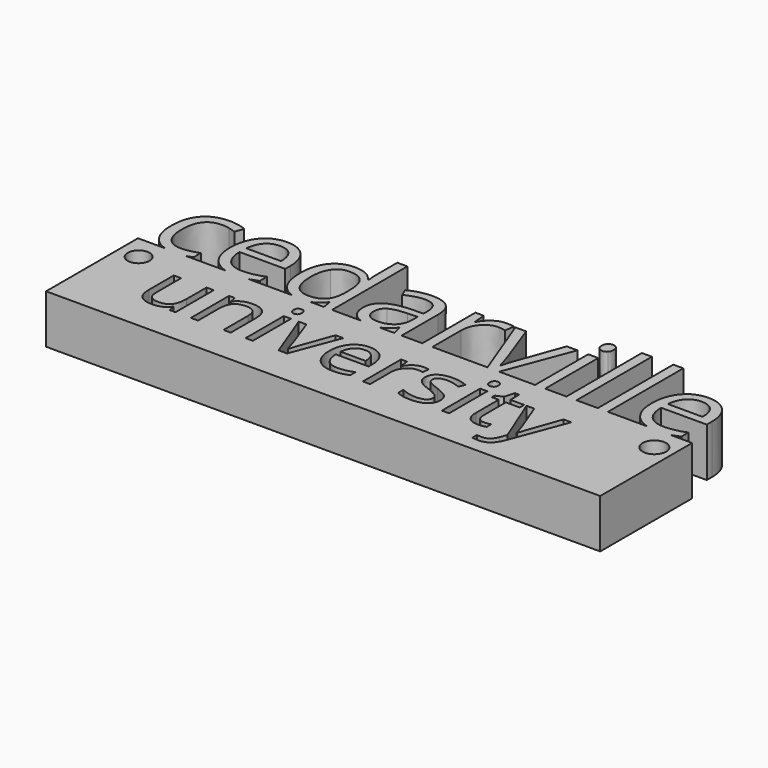
from build123d import *

# Parameters (mm, degrees)
F0_W         = 2.6162547147
F0_H         = 17.2652647355
F0_H_2       = 24.5141554478
F1_DEPTH     = 12.7
F2_R         = 2.841361974
F2_R_2       = 3.060651004
F3_DEPTH     = 25.4
F4_TEXT_SIZE = 23.2007315386
F5_DEPTH     = 72.644


# Not quite as in the source:
# - Text() gives the source's letters only with a copy of the font that has no kerning and outlines rounded to 1/6400 em; it was checked with that copy


with BuildPart() as f1:
    # F0 (on Top) → F1 (new body)
    with BuildSketch(Plane.XY):
        with BuildLine():
            Line((-23.2760247454, 28.446094293), (-22.9281989741, 26.1322967708))
            Line((-22.9281989741, 26.1322967708), (-20.8009167206, 26.1322967708))
            Line((-20.8009167206, 26.1322967708), (-20.8009167206, 50.6464522186))
            Line((-20.8009167206, 50.6464522186), (-23.4171714352, 50.6464522186))
            Line((-23.4171714352, 50.6464522186), (-23.4171714352, 43.6193634475))
            Line((-23.4171714352, 43.6193634475), (-23.3516390435, 42.4044937245))
            Line((-23.3516390435, 42.4044937245), (-23.240738073, 41.1593782822))
            Line((-23.240738073, 41.1593782822), (-23.4474171545, 41.1593782822))
            add(Edge.make_bspline(
                [(-28.8361961332, 43.7151415584), (-25.3226517477, 43.7151415584), (-23.4474171545, 41.1593782822)],
                knots=[0, 0, 0, 1, 1, 1], degree=2))
            add(Edge.make_bspline(
                [(-34.0989512818, 41.3509345041), (-32.208593829, 43.7151415584), (-28.8361961332, 43.7151415584)],
                knots=[0, 0, 0, 1, 1, 1], degree=2))
            add(Edge.make_bspline(
                [(-35.9893087346, 34.7170400831), (-35.9893087346, 38.9867274498), (-34.0989512818, 41.3509345041)],
                knots=[0, 0, 0, 1, 1, 1], degree=2))
            add(Edge.make_bspline(
                [(-34.1065127116, 28.1310347176), (-35.9893087346, 30.4473527164), (-35.9893087346, 34.7170400831)],
                knots=[0, 0, 0, 1, 1, 1], degree=2))
            add(Edge.make_bspline(
                [(-31.138536455, 26.1322967708), (-32.9208740045, 26.6723975397), (-34.1065127116, 28.1310347176)],
                knots=[0.3702776654, 0.3702776654, 0.3702776654, 1, 1, 1], degree=2))
            Line((-31.138536455, 26.1322967708), (-26.5456043362, 26.1322967708))
            add(Edge.make_bspline(
                [(-23.4171714352, 28.446094293), (-24.5981755511, 26.7288682527), (-26.5456043362, 26.1322967708)],
                knots=[0, 0, 0, 0.6525958331, 0.6525958331, 0.6525958331], degree=2))
            Line((-23.4171714352, 28.446094293), (-23.2760247454, 28.446094293))
        make_face()
        with BuildLine():
            add(Edge.make_bspline(
                [(-28.5034932216, 28.007531364), (-25.8267470684, 28.007531364), (-24.6219592518, 29.4643668409)],
                knots=[0, 0, 0, 1, 1, 1], degree=2))
            add(Edge.make_bspline(
                [(-32.0649266626, 29.6937302119), (-30.8525774162, 28.007531364), (-28.5034932216, 28.007531364)],
                knots=[0, 0, 0, 1, 1, 1], degree=2))
            add(Edge.make_bspline(
                [(-33.277275909, 34.6867943639), (-33.277275909, 31.3799290598), (-32.0649266626, 29.6937302119)],
                knots=[0, 0, 0, 1, 1, 1], degree=2))
            add(Edge.make_bspline(
                [(-32.0573652328, 39.7353090011), (-33.277275909, 37.9482910891), (-33.277275909, 34.6867943639)],
                knots=[0, 0, 0, 1, 1, 1], degree=2))
            add(Edge.make_bspline(
                [(-28.5337389408, 41.5223269132), (-30.8374545566, 41.5223269132), (-32.0573652328, 39.7353090011)],
                knots=[0, 0, 0, 1, 1, 1], degree=2))
            add(Edge.make_bspline(
                [(-24.6370821114, 39.9545904656), (-25.8569927876, 41.5223269132), (-28.5337389408, 41.5223269132)],
                knots=[0, 0, 0, 1, 1, 1], degree=2))
            add(Edge.make_bspline(
                [(-23.4171714352, 34.7170400831), (-23.4171714352, 38.3868540181), (-24.6370821114, 39.9545904656)],
                knots=[0, 0, 0, 1, 1, 1], degree=2))
            Line((-23.4171714352, 34.7170400831), (-23.4171714352, 34.1675761835))
            add(Edge.make_bspline(
                [(-24.6219592518, 29.4643668409), (-23.4171714352, 30.9212023179), (-23.4171714352, 34.1675761835)],
                knots=[0, 0, 0, 1, 1, 1], degree=2))
        make_face(mode=Mode.SUBTRACT)
        with BuildLine():
            Line((-20.8009167206, 26.1322967708), (-22.9281989741, 26.1322967708))
            Line((-22.9281989741, 26.1322967708), (-26.5456043362, 26.1322967708))
            add(Edge.make_bspline(
                [(-26.5456043362, 26.1322967708), (-27.5823024583, 25.8147167187), (-28.8361961332, 25.8147167187)],
                knots=[0.6525958331, 0.6525958331, 0.6525958331, 1, 1, 1], degree=2))
            add(Edge.make_bspline(
                [(-28.8361961332, 25.8147167187), (-30.0905193361, 25.8147167187), (-31.138536455, 26.1322967708)],
                knots=[0, 0, 0, 0.3702776654, 0.3702776654, 0.3702776654], degree=2))
            Line((-31.138536455, 26.1322967708), (-42.60280741, 26.1322967708))
            add(Edge.make_bspline(
                [(-42.60280741, 26.1322967708), (-42.7271751485, 26.1029250075), (-42.85004605, 26.0768462855)],
                knots=[0.9005120931, 0.9005120931, 0.9005120931, 1, 1, 1], degree=2))
            add(Edge.make_bspline(
                [(-42.85004605, 26.0768462855), (-44.0850795858, 25.8147167187), (-45.8342903488, 25.8147167187)],
                knots=[0, 0, 0, 1, 1, 1], degree=2))
            add(Edge.make_bspline(
                [(-45.8342903488, 25.8147167187), (-47.2456387033, 25.8147167187), (-48.4378362443, 26.1322967708)],
                knots=[0, 0, 0, 0.3688754729, 0.3688754729, 0.3688754729], degree=2))
            Line((-48.4378362443, 26.1322967708), (-58.7826764594, 26.1322967708))
            add(Edge.make_bspline(
                [(-58.7826764594, 26.1322967708), (-60.0261827647, 25.8147167187), (-61.5872691221, 25.8147167187)],
                knots=[0.406741787, 0.406741787, 0.406741787, 1, 1, 1], degree=2))
            add(Edge.make_bspline(
                [(-61.5872691221, 25.8147167187), (-62.9782563342, 25.8147167187), (-64.1362590541, 26.1322967708)],
                knots=[0, 0, 0, 0.3708835197, 0.3708835197, 0.3708835197], degree=2))
            Line((-64.1362590541, 26.1322967708), (-71.2608583272, 26.1322967708))
            Line((-71.2608583272, 26.1322967708), (-71.2608583272, -3.7426400431))
            Line((-71.2608583272, -3.7426400431), (72.8596820975, -3.7426400431))
            Line((72.8596820975, -3.7426400431), (72.8596820975, 26.1322967708))
            Line((72.8596820975, 26.1322967708), (67.0278429456, 26.1322967708))
            add(Edge.make_bspline(
                [(67.0278429456, 26.1322967708), (66.9034752071, 26.1029250075), (66.7806043057, 26.0768462855)],
                knots=[0.9005120931, 0.9005120931, 0.9005120931, 1, 1, 1], degree=2))
            add(Edge.make_bspline(
                [(66.7806043057, 26.0768462855), (65.5455707699, 25.8147167187), (63.7963600069, 25.8147167187)],
                knots=[0, 0, 0, 1, 1, 1], degree=2))
            add(Edge.make_bspline(
                [(63.7963600069, 25.8147167187), (62.3850116524, 25.8147167187), (61.1928141113, 26.1322967708)],
                knots=[0, 0, 0, 0.3688754729, 0.3688754729, 0.3688754729], degree=2))
            Line((61.1928141113, 26.1322967708), (50.9570521875, 26.1322967708))
            Line((50.9570521875, 26.1322967708), (48.3407974728, 26.1322967708))
            Line((48.3407974728, 26.1322967708), (42.7957489446, 26.1322967708))
            Line((42.7957489446, 26.1322967708), (40.17949423, 26.1322967708))
            Line((40.17949423, 26.1322967708), (34.6344457018, 26.1322967708))
            Line((34.6344457018, 26.1322967708), (32.0181909871, 26.1322967708))
            Line((32.0181909871, 26.1322967708), (22.6924275533, 26.1322967708))
            Line((22.6924275533, 26.1322967708), (19.6376099096, 26.1322967708))
            Line((19.6376099096, 26.1322967708), (5.3011389876, 26.1322967708))
            Line((5.3011389876, 26.1322967708), (2.6848842729, 26.1322967708))
            Line((2.6848842729, 26.1322967708), (-2.6988537526, 26.1322967708))
            Line((-2.6988537526, 26.1322967708), (-4.6396207375, 26.1322967708))
            Line((-4.6396207375, 26.1322967708), (-8.5637145698, 26.1322967708))
            add(Edge.make_bspline(
                [(-8.5637145698, 26.1322967708), (-9.6384567354, 25.8147167187), (-11.066836077, 25.8147167187)],
                knots=[0.2582329607, 0.2582329607, 0.2582329607, 1, 1, 1], degree=2))
            add(Edge.make_bspline(
                [(-11.066836077, 25.8147167187), (-12.3226429307, 25.8147167187), (-13.3127934671, 26.1322967708)],
                knots=[0, 0, 0, 0.4894320446, 0.4894320446, 0.4894320446], degree=2))
            Line((-13.3127934671, 26.1322967708), (-20.8009167206, 26.1322967708))
        make_face()
        with BuildLine():
            add(Edge.make_bspline(
                [(-26.5456043362, 26.1322967708), (-27.5823024583, 25.8147167187), (-28.8361961332, 25.8147167187)],
                knots=[0.6525958331, 0.6525958331, 0.6525958331, 1, 1, 1], degree=2))
            Line((-26.5456043362, 26.1322967708), (-31.138536455, 26.1322967708))
            add(Edge.make_bspline(
                [(-28.8361961332, 25.8147167187), (-30.0905193361, 25.8147167187), (-31.138536455, 26.1322967708)],
                knots=[0, 0, 0, 0.3702776654, 0.3702776654, 0.3702776654], degree=2))
        make_face()
        with BuildLine():
            add(Edge.make_bspline(
                [(-13.3127934671, 26.1322967708), (-14.3457032256, 26.4635913799), (-15.0895167365, 27.1404874123)],
                knots=[0.4894320446, 0.4894320446, 0.4894320446, 1, 1, 1], degree=2))
            Line((-13.3127934671, 26.1322967708), (-8.5637145698, 26.1322967708))
            add(Edge.make_bspline(
                [(-7.8582693604, 26.391905861), (-8.1895622595, 26.2428565999), (-8.5637145698, 26.1322967708)],
                knots=[0, 0, 0, 0.2582329607, 0.2582329607, 0.2582329607], degree=2))
            add(Edge.make_bspline(
                [(-5.284862748, 28.592281936), (-6.5753467691, 26.9690950032), (-7.8582693604, 26.391905861)],
                knots=[0, 0, 0, 1, 1, 1], degree=2))
            Line((-5.284862748, 28.592281936), (-5.1588389179, 28.592281936))
            Line((-5.1588389179, 28.592281936), (-4.6396207375, 26.1322967708))
            Line((-4.6396207375, 26.1322967708), (-2.6988537526, 26.1322967708))
            Line((-2.6988537526, 26.1322967708), (-2.6988537526, 37.9180453698))
            add(Edge.make_bspline(
                [(-4.1884554254, 42.3112360901), (-2.6988537526, 40.9426172943), (-2.6988537526, 37.9180453698)],
                knots=[0, 0, 0, 1, 1, 1], degree=2))
            add(Edge.make_bspline(
                [(-8.7631204612, 43.6798548859), (-5.6780570982, 43.6798548859), (-4.1884554254, 42.3112360901)],
                knots=[0, 0, 0, 1, 1, 1], degree=2))
            add(Edge.make_bspline(
                [(-11.8154176283, 43.2866605358), (-10.2955702362, 43.6798548859), (-8.7631204612, 43.6798548859)],
                knots=[0, 0, 0, 1, 1, 1], degree=2))
            add(Edge.make_bspline(
                [(-14.6106261818, 42.2028555962), (-13.3352650203, 42.8934661856), (-11.8154176283, 43.2866605358)],
                knots=[0, 0, 0, 1, 1, 1], degree=2))
            Line((-14.6106261818, 42.2028555962), (-13.8040736686, 40.2015971728))
            add(Edge.make_bspline(
                [(-8.9244309638, 41.5223269132), (-11.0819589366, 41.5223269132), (-13.8040736686, 40.2015971728)],
                knots=[0, 0, 0, 1, 1, 1], degree=2))
            add(Edge.make_bspline(
                [(-6.1267019337, 40.5544638973), (-6.9987868386, 41.5223269132), (-8.9244309638, 41.5223269132)],
                knots=[0, 0, 0, 1, 1, 1], degree=2))
            add(Edge.make_bspline(
                [(-5.2546170288, 37.5550967389), (-5.2546170288, 39.5866008815), (-6.1267019337, 40.5544638973)],
                knots=[0, 0, 0, 1, 1, 1], degree=2))
            Line((-5.2546170288, 37.5550967389), (-5.2546170288, 36.4813737057))
            Line((-5.2546170288, 36.4813737057), (-8.1834108423, 36.3855955948))
            add(Edge.make_bspline(
                [(-16.5463522135, 30.9060794583), (-16.5463522135, 36.1335479344), (-8.1834108423, 36.3855955948)],
                knots=[0, 0, 0, 1, 1, 1], degree=2))
            add(Edge.make_bspline(
                [(-15.0895167365, 27.1404874123), (-16.5463522135, 28.4662581059), (-16.5463522135, 30.9060794583)],
                knots=[0, 0, 0, 1, 1, 1], degree=2))
        make_face()
        with BuildLine():
            add(Edge.make_bspline(
                [(-10.5476178966, 27.9772856447), (-8.102755591, 27.9772856447), (-6.7089320291, 29.3156587213)],
                knots=[0, 0, 0, 1, 1, 1], degree=2))
            add(Edge.make_bspline(
                [(-12.9471116234, 28.7157852896), (-12.0901495781, 27.9772856447), (-10.5476178966, 27.9772856447)],
                knots=[0, 0, 0, 1, 1, 1], degree=2))
            add(Edge.make_bspline(
                [(-13.8040736686, 30.875833739), (-13.8040736686, 29.4542849345), (-12.9471116234, 28.7157852896)],
                knots=[0, 0, 0, 1, 1, 1], degree=2))
            add(Edge.make_bspline(
                [(-12.427893443, 33.5450184624), (-13.8040736686, 32.6855359405), (-13.8040736686, 30.875833739)],
                knots=[0, 0, 0, 1, 1, 1], degree=2))
            add(Edge.make_bspline(
                [(-7.9313631819, 34.5154019548), (-11.0517132174, 34.4045009842), (-12.427893443, 33.5450184624)],
                knots=[0, 0, 0, 1, 1, 1], degree=2))
            Line((-7.9313631819, 34.5154019548), (-5.3151084673, 34.6212619722))
            Line((-5.3151084673, 34.6212619722), (-5.3151084673, 33.0636074311))
            add(Edge.make_bspline(
                [(-6.7089320291, 29.3156587213), (-5.3151084673, 30.6540317979), (-5.3151084673, 33.0636074311)],
                knots=[0, 0, 0, 1, 1, 1], degree=2))
        make_face(mode=Mode.SUBTRACT)
        with BuildLine():
            Line((-8.5637145698, 26.1322967708), (-13.3127934671, 26.1322967708))
            add(Edge.make_bspline(
                [(-11.066836077, 25.8147167187), (-12.3226429307, 25.8147167187), (-13.3127934671, 26.1322967708)],
                knots=[0, 0, 0, 0.4894320446, 0.4894320446, 0.4894320446], degree=2))
            add(Edge.make_bspline(
                [(-8.5637145698, 26.1322967708), (-9.6384567354, 25.8147167187), (-11.066836077, 25.8147167187)],
                knots=[0.2582329607, 0.2582329607, 0.2582329607, 1, 1, 1], degree=2))
        make_face()
        with BuildLine():
            add(Edge.make_bspline(
                [(-42.60280741, 26.1322967708), (-42.7271751485, 26.1029250075), (-42.85004605, 26.0768462855)],
                knots=[0.9005120931, 0.9005120931, 0.9005120931, 1, 1, 1], degree=2))
            Line((-42.60280741, 26.1322967708), (-48.4378362443, 26.1322967708))
            add(Edge.make_bspline(
                [(-45.8342903488, 25.8147167187), (-47.2456387033, 25.8147167187), (-48.4378362443, 26.1322967708)],
                knots=[0, 0, 0, 0.3688754729, 0.3688754729, 0.3688754729], degree=2))
            add(Edge.make_bspline(
                [(-42.85004605, 26.0768462855), (-44.0850795858, 25.8147167187), (-45.8342903488, 25.8147167187)],
                knots=[0, 0, 0, 1, 1, 1], degree=2))
        make_face()
        with BuildLine():
            Line((-48.4378362443, 26.1322967708), (-42.60280741, 26.1322967708))
            add(Edge.make_bspline(
                [(-40.2287503821, 26.9338083308), (-41.4770961962, 26.3981544906), (-42.60280741, 26.1322967708)],
                knots=[0, 0, 0, 0.9005120931, 0.9005120931, 0.9005120931], degree=2))
            Line((-40.2287503821, 26.9338083308), (-40.2287503821, 29.2677696658))
            add(Edge.make_bspline(
                [(-45.7385122378, 28.1033094749), (-42.9508651141, 28.1033094749), (-40.2287503821, 29.2677696658)],
                knots=[0, 0, 0, 1, 1, 1], degree=2))
            add(Edge.make_bspline(
                [(-49.8418481487, 29.6786073523), (-48.3850126717, 28.1033094749), (-45.7385122378, 28.1033094749)],
                knots=[0, 0, 0, 1, 1, 1], degree=2))
            add(Edge.make_bspline(
                [(-51.379338877, 34.2936000137), (-51.2986836256, 31.2539052296), (-49.8418481487, 29.6786073523)],
                knots=[0, 0, 0, 1, 1, 1], degree=2))
            Line((-51.379338877, 34.2936000137), (-39.4877302606, 34.2936000137))
            Line((-39.4877302606, 34.2936000137), (-39.4877302606, 35.9470326657))
            add(Edge.make_bspline(
                [(-41.3780877134, 41.580297875), (-39.4877302606, 39.4454541917), (-39.4877302606, 35.9470326657)],
                knots=[0, 0, 0, 1, 1, 1], degree=2))
            add(Edge.make_bspline(
                [(-46.5097780786, 43.7151415584), (-43.2684451662, 43.7151415584), (-41.3780877134, 41.580297875)],
                knots=[0, 0, 0, 1, 1, 1], degree=2))
            add(Edge.make_bspline(
                [(-52.0346627939, 41.2576768698), (-49.9779538853, 43.7151415584), (-46.5097780786, 43.7151415584)],
                knots=[0, 0, 0, 1, 1, 1], degree=2))
            add(Edge.make_bspline(
                [(-54.0913717026, 34.6212619722), (-54.0913717026, 38.8002121811), (-52.0346627939, 41.2576768698)],
                knots=[0, 0, 0, 1, 1, 1], degree=2))
            add(Edge.make_bspline(
                [(-51.8758727679, 28.1486780538), (-54.0913717026, 30.4826393888), (-54.0913717026, 34.6212619722)],
                knots=[0, 0, 0, 1, 1, 1], degree=2))
            add(Edge.make_bspline(
                [(-48.4378362443, 26.1322967708), (-50.4776170504, 26.6756578098), (-51.8758727679, 28.1486780538)],
                knots=[0.3688754729, 0.3688754729, 0.3688754729, 1, 1, 1], degree=2))
        make_face()
        with BuildLine():
            add(Edge.make_bspline(
                [(-46.545064751, 41.5223269132), (-48.6219374725, 41.5223269132), (-49.8594914849, 40.168830977)],
                knots=[0, 0, 0, 1, 1, 1], degree=2))
            add(Edge.make_bspline(
                [(-43.3919485198, 40.206638126), (-44.4933967956, 41.5223269132), (-46.545064751, 41.5223269132)],
                knots=[0, 0, 0, 1, 1, 1], degree=2))
            add(Edge.make_bspline(
                [(-42.2905002439, 36.4208822672), (-42.2905002439, 38.8909493389), (-43.3919485198, 40.206638126)],
                knots=[0, 0, 0, 1, 1, 1], degree=2))
            Line((-42.2905002439, 36.4208822672), (-51.3188474385, 36.4208822672))
            add(Edge.make_bspline(
                [(-49.8594914849, 40.168830977), (-51.0970454973, 38.8153350408), (-51.3188474385, 36.4208822672)],
                knots=[0, 0, 0, 1, 1, 1], degree=2))
        make_face(mode=Mode.SUBTRACT)
        with BuildLine():
            add(Edge.make_bspline(
                [(-58.7826764594, 26.1322967708), (-60.0261827647, 25.8147167187), (-61.5872691221, 25.8147167187)],
                knots=[0.406741787, 0.406741787, 0.406741787, 1, 1, 1], degree=2))
            Line((-58.7826764594, 26.1322967708), (-64.1362590541, 26.1322967708))
            add(Edge.make_bspline(
                [(-61.5872691221, 25.8147167187), (-62.9782563342, 25.8147167187), (-64.1362590541, 26.1322967708)],
                knots=[0, 0, 0, 0.3708835197, 0.3708835197, 0.3708835197], degree=2))
        make_face()
        with BuildLine():
            Line((-64.1362590541, 26.1322967708), (-58.7826764594, 26.1322967708))
            add(Edge.make_bspline(
                [(-57.2268445976, 26.7170473429), (-57.930120244, 26.3500317723), (-58.7826764594, 26.1322967708)],
                knots=[0, 0, 0, 0.406741787, 0.406741787, 0.406741787], degree=2))
            Line((-57.2268445976, 26.7170473429), (-57.2268445976, 29.0308448651))
            add(Edge.make_bspline(
                [(-61.6528015137, 28.1033094749), (-59.495273541, 28.1033094749), (-57.2268445976, 29.0308448651)],
                knots=[0, 0, 0, 1, 1, 1], degree=2))
            add(Edge.make_bspline(
                [(-65.4562007088, 29.8046311824), (-64.1732781175, 28.1033094749), (-61.6528015137, 28.1033094749)],
                knots=[0, 0, 0, 1, 1, 1], degree=2))
            add(Edge.make_bspline(
                [(-66.7391233001, 34.6867943639), (-66.7391233001, 31.50595289), (-65.4562007088, 29.8046311824)],
                knots=[0, 0, 0, 1, 1, 1], degree=2))
            add(Edge.make_bspline(
                [(-61.4763681515, 41.396303083), (-66.7391233001, 41.396303083), (-66.7391233001, 34.6867943639)],
                knots=[0, 0, 0, 1, 1, 1], degree=2))
            add(Edge.make_bspline(
                [(-59.66666595, 41.1694601886), (-60.6899794511, 41.396303083), (-61.4763681515, 41.396303083)],
                knots=[0, 0, 0, 1, 1, 1], degree=2))
            add(Edge.make_bspline(
                [(-57.7763084972, 40.594791523), (-58.6433524489, 40.9426172943), (-59.66666595, 41.1694601886)],
                knots=[0, 0, 0, 1, 1, 1], degree=2))
            Line((-57.7763084972, 40.594791523), (-56.9747969372, 42.8128109343))
            add(Edge.make_bspline(
                [(-58.9256458285, 43.4454505618), (-57.6805303863, 43.1757595652), (-56.9747969372, 42.8128109343)],
                knots=[0, 0, 0, 1, 1, 1], degree=2))
            add(Edge.make_bspline(
                [(-61.415876713, 43.7151415584), (-60.1707612708, 43.7151415584), (-58.9256458285, 43.4454505618)],
                knots=[0, 0, 0, 1, 1, 1], degree=2))
            add(Edge.make_bspline(
                [(-67.3616810212, 41.3509345041), (-65.2722059167, 43.7151415584), (-61.415876713, 43.7151415584)],
                knots=[0, 0, 0, 1, 1, 1], degree=2))
            add(Edge.make_bspline(
                [(-69.4511561257, 34.6565486446), (-69.4511561257, 38.9867274498), (-67.3616810212, 41.3509345041)],
                knots=[0, 0, 0, 1, 1, 1], degree=2))
            add(Edge.make_bspline(
                [(-67.394447217, 28.1234732878), (-69.4511561257, 30.4322298568), (-69.4511561257, 34.6565486446)],
                knots=[0, 0, 0, 1, 1, 1], degree=2))
            add(Edge.make_bspline(
                [(-64.1362590541, 26.1322967708), (-66.1005377473, 26.6709964811), (-67.394447217, 28.1234732878)],
                knots=[0.3708835197, 0.3708835197, 0.3708835197, 1, 1, 1], degree=2))
        make_face()
        with BuildLine():
            Line((2.6848842729, 43.3975615063), (2.6848842729, 26.1322967708))
            Line((2.6848842729, 26.1322967708), (5.3011389876, 26.1322967708))
            Line((5.3011389876, 26.1322967708), (5.3011389876, 35.3975687661))
            add(Edge.make_bspline(
                [(6.7882201838, 39.634489937), (5.3011389876, 37.9331682295), (5.3011389876, 35.3975687661)],
                knots=[0, 0, 0, 1, 1, 1], degree=2))
            add(Edge.make_bspline(
                [(10.3723379143, 41.3358116445), (8.27530138, 41.3358116445), (6.7882201838, 39.634489937)],
                knots=[0, 0, 0, 1, 1, 1], degree=2))
            add(Edge.make_bspline(
                [(12.2626953671, 41.0988868437), (11.1940132871, 41.3358116445), (10.3723379143, 41.3358116445)],
                knots=[0, 0, 0, 1, 1, 1], degree=2))
            Line((12.2626953671, 41.0988868437), (12.625643998, 43.5235853365))
            add(Edge.make_bspline(
                [(10.5638941362, 43.7151415584), (11.7132314675, 43.7151415584), (12.625643998, 43.5235853365)],
                knots=[0, 0, 0, 1, 1, 1], degree=2))
            add(Edge.make_bspline(
                [(7.5846907906, 42.8002085512), (8.9407072034, 43.7151415584), (10.5638941362, 43.7151415584)],
                knots=[0, 0, 0, 1, 1, 1], degree=2))
            add(Edge.make_bspline(
                [(5.2708932684, 40.2015971728), (6.2286743778, 41.8852755441), (7.5846907906, 42.8002085512)],
                knots=[0, 0, 0, 1, 1, 1], degree=2))
            Line((5.2708932684, 40.2015971728), (5.1448694382, 40.2015971728))
            Line((5.1448694382, 40.2015971728), (4.8424122457, 43.3975615063))
            Line((4.8424122457, 43.3975615063), (2.6848842729, 43.3975615063))
        make_face()
        with BuildLine():
            Line((13.0843707399, 43.3975615063), (19.6376099096, 26.1322967708))
            Line((19.6376099096, 26.1322967708), (22.6924275533, 26.1322967708))
            Line((22.6924275533, 26.1322967708), (29.245666723, 43.3975615063))
            Line((29.245666723, 43.3975615063), (26.4428967397, 43.3975615063))
            add(Edge.make_bspline(
                [(22.3093151095, 31.9520772488), (23.2318095465, 34.5758933933), (26.4428967397, 43.3975615063)],
                knots=[0, 0, 0, 1, 1, 1], degree=2))
            add(Edge.make_bspline(
                [(21.2154282635, 28.4965038251), (21.3868206726, 29.3282611043), (22.3093151095, 31.9520772488)],
                knots=[0, 0, 0, 1, 1, 1], degree=2))
            Line((21.2154282635, 28.4965038251), (21.0894044333, 28.4965038251))
            add(Edge.make_bspline(
                [(19.6073641904, 33.159385542), (20.8676024922, 29.5651859051), (21.0894044333, 28.4965038251)],
                knots=[0, 0, 0, 1, 1, 1], degree=2))
            Line((19.6073641904, 33.159385542), (15.8871407233, 43.3975615063))
            Line((15.8871407233, 43.3975615063), (13.0843707399, 43.3975615063))
        make_face()
        with Locations((33.3263183444, 34.7649291386)):
            Rectangle(F0_W, F0_H)
        with BuildLine():
            add(Edge.make_bspline(
                [(67.0278429456, 26.1322967708), (66.9034752071, 26.1029250075), (66.7806043057, 26.0768462855)],
                knots=[0.9005120931, 0.9005120931, 0.9005120931, 1, 1, 1], degree=2))
            Line((67.0278429456, 26.1322967708), (61.1928141113, 26.1322967708))
            add(Edge.make_bspline(
                [(63.7963600069, 25.8147167187), (62.3850116524, 25.8147167187), (61.1928141113, 26.1322967708)],
                knots=[0, 0, 0, 0.3688754729, 0.3688754729, 0.3688754729], degree=2))
            add(Edge.make_bspline(
                [(66.7806043057, 26.0768462855), (65.5455707699, 25.8147167187), (63.7963600069, 25.8147167187)],
                knots=[0, 0, 0, 1, 1, 1], degree=2))
        make_face()
        with BuildLine():
            Line((61.1928141113, 26.1322967708), (67.0278429456, 26.1322967708))
            add(Edge.make_bspline(
                [(69.4018999736, 26.9338083308), (68.1535541595, 26.3981544906), (67.0278429456, 26.1322967708)],
                knots=[0, 0, 0, 0.9005120931, 0.9005120931, 0.9005120931], degree=2))
            Line((69.4018999736, 26.9338083308), (69.4018999736, 29.2677696658))
            add(Edge.make_bspline(
                [(63.8921381178, 28.1033094749), (66.6797852415, 28.1033094749), (69.4018999736, 29.2677696658)],
                knots=[0, 0, 0, 1, 1, 1], degree=2))
            add(Edge.make_bspline(
                [(59.7888022069, 29.6786073523), (61.2456376839, 28.1033094749), (63.8921381178, 28.1033094749)],
                knots=[0, 0, 0, 1, 1, 1], degree=2))
            add(Edge.make_bspline(
                [(58.2513114787, 34.2936000137), (58.33196673, 31.2539052296), (59.7888022069, 29.6786073523)],
                knots=[0, 0, 0, 1, 1, 1], degree=2))
            Line((58.2513114787, 34.2936000137), (70.142920095, 34.2936000137))
            Line((70.142920095, 34.2936000137), (70.142920095, 35.9470326657))
            add(Edge.make_bspline(
                [(68.2525626423, 41.580297875), (70.142920095, 39.4454541917), (70.142920095, 35.9470326657)],
                knots=[0, 0, 0, 1, 1, 1], degree=2))
            add(Edge.make_bspline(
                [(63.1208722771, 43.7151415584), (66.3622051895, 43.7151415584), (68.2525626423, 41.580297875)],
                knots=[0, 0, 0, 1, 1, 1], degree=2))
            add(Edge.make_bspline(
                [(57.5959875617, 41.2576768698), (59.6526964703, 43.7151415584), (63.1208722771, 43.7151415584)],
                knots=[0, 0, 0, 1, 1, 1], degree=2))
            add(Edge.make_bspline(
                [(55.5392786531, 34.6212619722), (55.5392786531, 38.8002121811), (57.5959875617, 41.2576768698)],
                knots=[0, 0, 0, 1, 1, 1], degree=2))
            add(Edge.make_bspline(
                [(57.7547775877, 28.1486780538), (55.5392786531, 30.4826393888), (55.5392786531, 34.6212619722)],
                knots=[0, 0, 0, 1, 1, 1], degree=2))
            add(Edge.make_bspline(
                [(61.1928141113, 26.1322967708), (59.1530333053, 26.6756578098), (57.7547775877, 28.1486780538)],
                knots=[0.3688754729, 0.3688754729, 0.3688754729, 1, 1, 1], degree=2))
        make_face()
        with BuildLine():
            add(Edge.make_bspline(
                [(63.0855856046, 41.5223269132), (61.0087128831, 41.5223269132), (59.7711588707, 40.168830977)],
                knots=[0, 0, 0, 1, 1, 1], degree=2))
            add(Edge.make_bspline(
                [(66.2387018359, 40.206638126), (65.13725356, 41.5223269132), (63.0855856046, 41.5223269132)],
                knots=[0, 0, 0, 1, 1, 1], degree=2))
            add(Edge.make_bspline(
                [(67.3401501117, 36.4208822672), (67.3401501117, 38.8909493389), (66.2387018359, 40.206638126)],
                knots=[0, 0, 0, 1, 1, 1], degree=2))
            Line((67.3401501117, 36.4208822672), (58.3118029172, 36.4208822672))
            add(Edge.make_bspline(
                [(59.7711588707, 40.168830977), (58.5336048583, 38.8153350408), (58.3118029172, 36.4208822672)],
                knots=[0, 0, 0, 1, 1, 1], degree=2))
        make_face(mode=Mode.SUBTRACT)
        with Locations((41.4876215873, 38.3893744947)):
            Rectangle(F0_W, F0_H_2)
        with Locations((49.6489248302, 38.3893744947)):
            Rectangle(F0_W, F0_H_2)
        with BuildLine():
            add(Edge.make_bspline(
                [(31.796389046, 48.0755660828), (31.796389046, 48.9728557538), (32.2374724516, 49.39125487)],
                knots=[0, 0, 0, 1, 1, 1], degree=2))
            add(Edge.make_bspline(
                [(32.2374724516, 46.7598772957), (31.796389046, 47.1933992715), (31.796389046, 48.0755660828)],
                knots=[0, 0, 0, 1, 1, 1], degree=2))
            add(Edge.make_bspline(
                [(33.3439616807, 46.3263553199), (32.6785558573, 46.3263553199), (32.2374724516, 46.7598772957)],
                knots=[0, 0, 0, 1, 1, 1], degree=2))
            add(Edge.make_bspline(
                [(34.4302870969, 46.7598772957), (33.9740808316, 46.3263553199), (33.3439616807, 46.3263553199)],
                knots=[0, 0, 0, 1, 1, 1], degree=2))
            add(Edge.make_bspline(
                [(34.8864933621, 48.0755660828), (34.8864933621, 47.1933992715), (34.4302870969, 46.7598772957)],
                knots=[0, 0, 0, 1, 1, 1], degree=2))
            add(Edge.make_bspline(
                [(34.4302870969, 49.3836934402), (34.8864933621, 48.9577328941), (34.8864933621, 48.0755660828)],
                knots=[0, 0, 0, 1, 1, 1], degree=2))
            add(Edge.make_bspline(
                [(33.3439616807, 49.8096539862), (33.9740808316, 49.8096539862), (34.4302870969, 49.3836934402)],
                knots=[0, 0, 0, 1, 1, 1], degree=2))
            add(Edge.make_bspline(
                [(32.2374724516, 49.39125487), (32.6785558573, 49.8096539862), (33.3439616807, 49.8096539862)],
                knots=[0, 0, 0, 1, 1, 1], degree=2))
        make_face()
    extrude(amount=F1_DEPTH)

    # F2 (on Top) → F3 (cut)
    with BuildSketch(Plane.XY):
        with Locations((-66.0497844219, 19.8396835476)):
            Circle(F2_R)
        with Locations((68.0730268359, 19.8396835476)):
            Circle(F2_R_2)
    extrude(amount=F3_DEPTH, mode=Mode.SUBTRACT)

    # F4 (on face) → F5 (cut)
    with BuildSketch(Plane.XY.offset(12.7)):
        with Locations((-57.2268445976, 5.4814816592)):
            Text('university', F4_TEXT_SIZE, font='Open Sans', text_align=(TextAlign.LEFT, TextAlign.BOTTOM))
    extrude(amount=-F5_DEPTH, mode=Mode.SUBTRACT)


solid = f1.part
